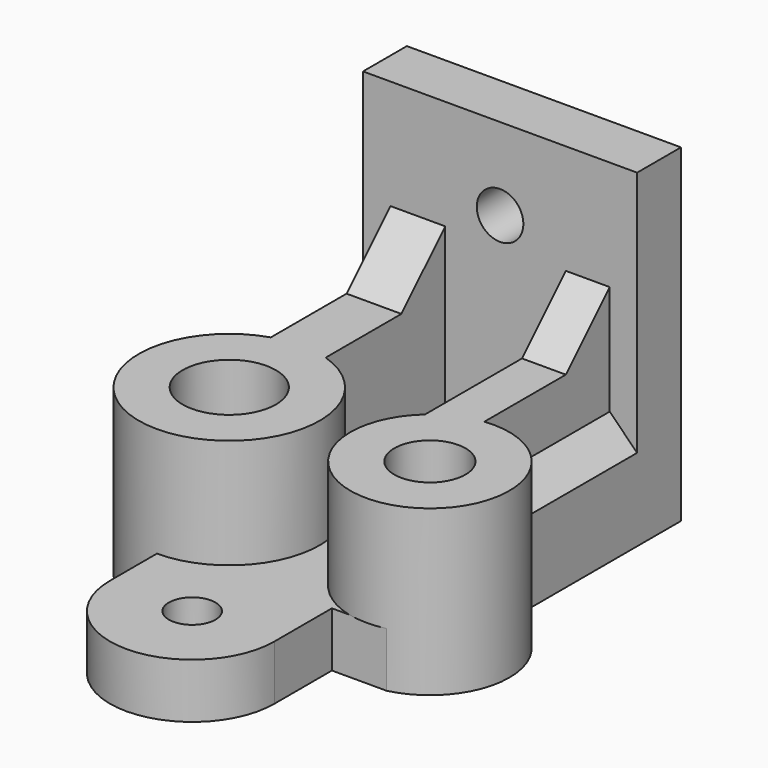
from build123d import *

# Parameters (mm, degrees)
F0_R          = 2.125
F0_R_2        = 4.25
F0_R_3        = 3.25
F1_DEPTH      = 5
F2_W          = 25
F2_H          = 5
F3_DEPTH      = 25
F4_R          = 8.25
F4_R_2        = 4.25
F4_R_3        = 7.25
F4_R_4        = 3.25
F5_DEPTH      = 10
F6_R          = 2.125
F7_DEPTH      = 5.001
F8_W          = 5
F8_H          = 13.6379074032
F8_W_2        = 4
F8_H_2        = 16.0665388563
F9_DEPTH      = 10
F10_T1_DEPTH  = 5
F10_T3_DEPTH  = 4
F10_T8_DEPTH  = 17.8584149398
F10_T13_DEPTH = 16.8584149398
F10_T18_DEPTH = 26.4963223431
F10_S19_R     = 8.25
F10_T20_DEPTH = 15
F10_T25_DEPTH = 26.4963223431
F10_S26_R     = 8.25
F10_T27_DEPTH = 15
F10_T32_DEPTH = 27.1526880508
F10_S34_R     = 7.25
F10_T35_DEPTH = 16


# Not quite as in the source:
# - a fillet or chamfer that OpenCascade refuses, or shapes differently, is made with other operations: its cross-section is extruded or revolved along the edge and cut away or added


with BuildPart() as f1:
    # F0 (on Top) → F1 (new body)
    with BuildSketch(Plane.XY):
        with BuildLine():
            Line((12.5, 26.5), (0, 26.5))
            Line((0, 26.5), (-12.5, 26.5))
            Line((-12.5, 26.5), (-12.5, 6.5622023742))
            ThreePointArc((-12.5, 6.5622023742), (-15.3166703137, -2.6385915194), (-7.5, -8.25))
            Line((-7.5, -8.25), (-7.5, -13.6))
            ThreePointArc((-7.5, -13.6), (-5.3033008589, -18.9033008589), (0, -21.1))
            ThreePointArc((0, -21.1), (5.3033008589, -18.9033008589), (7.5, -13.6))
            Line((7.5, -13.6), (7.5, -7.0478720193))
            Line((7.5, -7.0478720193), (12.5, -7.0478720193))
            ThreePointArc((12.5, -7.0478720193), (18.05, 0), (12.5, 7.0478720193))
            Line((12.5, 7.0478720193), (12.5, 26.5))
        make_face()
        with Locations((0, -13.6)):
            Circle(F0_R, mode=Mode.SUBTRACT)
        with Locations((-7.5, 0)):
            Circle(F0_R_2, mode=Mode.SUBTRACT)
        with Locations((10.8, 0)):
            Circle(F0_R_3, mode=Mode.SUBTRACT)
        with Locations((0, 16.5)):
            Circle(F0_R, mode=Mode.SUBTRACT)
    extrude(amount=F1_DEPTH)

    # F2 (on face) → F3 (join)
    with BuildSketch(Plane.XY.offset(5)):
        with Locations((0, 24)):
            Rectangle(F2_W, F2_H)
    extrude(amount=F3_DEPTH)

    # F4 (on face) → F5 (join)
    with BuildSketch(Plane.XY.offset(5)):
        with Locations((-7.5, 0)):
            Circle(F4_R)
        with Locations((-7.5, 0)):
            Circle(F4_R_2, mode=Mode.SUBTRACT)
        with Locations((10.8, 0)):
            Circle(F4_R_3)
        with Locations((10.8, 0)):
            Circle(F4_R_4, mode=Mode.SUBTRACT)
    extrude(amount=F5_DEPTH)

    # F6 (on face) → F7 (cut, through all)
    with BuildSketch(Plane.XZ.offset(-21.5)):
        with Locations((0, 22.5)):
            Circle(F6_R)
    extrude(amount=-F7_DEPTH, mode=Mode.SUBTRACT)

    # F8 (on face) → F9 (join)
    with BuildSketch(Plane.XY.offset(5)):
        with Locations((-7.5, 14.6810462984)):
            Rectangle(F8_W, F8_H)
        with Locations((8, 13.4667305718)):
            Rectangle(F8_W_2, F8_H_2)
    extrude(amount=F9_DEPTH)

    # F10: chamfer of 5 on 4 edges, made by hand

    # F10_s2 → F10_t1 (join)
    with BuildSketch(Plane.YZ.offset(-10)):
        Polygon((16.5, 15), (21.5, 20), (21.5, 15), align=None)
    extrude(amount=F10_T1_DEPTH)

    # F10_s4 → F10_t3 (join)
    with BuildSketch(Plane.YZ.offset(6)):
        Polygon((16.5, 15), (21.5, 20), (21.5, 15), align=None)
    extrude(amount=F10_T3_DEPTH)


with BuildPart() as f10_tool6:
    # F10_s7 → F10_t8 (new body)
    with BuildSketch(Plane.YZ.offset(7.8584149398)):
        Polygon((16.5, 15), (21.5, 20), (21.5, 15), align=None)
    extrude(amount=-F10_T8_DEPTH)

    split(bisect_by=Plane.YZ.offset(6), keep=Keep.TOP)


with BuildPart() as f1_1:
    add(f1.part)

    # F10_t5: union F10_tool6
    add(f10_tool6.part)


with BuildPart() as f10_tool11:
    # F10_s12 → F10_t13 (new body)
    with BuildSketch(Plane.YZ.offset(10)):
        Polygon((16.5, 15), (21.5, 20), (21.5, 15), align=None)
    extrude(amount=-F10_T13_DEPTH)

    split(bisect_by=Plane.YZ.offset(-5), keep=Keep.BOTTOM)


with BuildPart() as f1_2:
    add(f1_1.part)

    # F10_t10: union F10_tool11
    add(f10_tool11.part)


with BuildPart() as f10_tool16:
    # F10_s17 → F10_t18 (new body)
    with BuildSketch(Plane.XZ.offset(-21.5)):
        Polygon((-10, 10), (-15, 5), (-10, 5), align=None)
    extrude(amount=F10_T18_DEPTH)

    # F10_s19 → F10_t20 (cut, symmetric)
    with BuildSketch(Plane.XY.offset(7.5)):
        with Locations((-7.5, 0)):
            Circle(F10_S19_R)
    extrude(amount=F10_T20_DEPTH, both=True, mode=Mode.SUBTRACT)

    split(bisect_by=Plane.YZ.offset(-12.5), keep=Keep.TOP)


with BuildPart() as f1_3:
    add(f1_2.part)

    # F10_t15: union F10_tool16
    add(f10_tool16.part)


with BuildPart() as f10_tool23:
    # F10_s24 → F10_t25 (new body)
    with BuildSketch(Plane.XZ.offset(-21.5)):
        Polygon((-10, 10), (-15, 5), (-10, 5), align=None)
    extrude(amount=F10_T25_DEPTH)

    # F10_s26 → F10_t27 (intersect, symmetric)
    with BuildSketch(Plane.XY.offset(7.5)):
        with Locations((-7.5, 0)):
            Circle(F10_S26_R)
    extrude(amount=F10_T27_DEPTH, both=True, mode=Mode.INTERSECT)

    split(bisect_by=Plane.YZ.offset(-12.5), keep=Keep.BOTTOM)


with BuildPart() as f1_4:
    add(f1_3.part)

    # F10_t22: union F10_tool23
    add(f10_tool23.part)


with BuildPart() as f10_tool30:
    # F10_s31 → F10_t32 (new body)
    with BuildSketch(Plane.XZ.offset(5.6526880508)):
        Polygon((10, 10), (15, 5), (10, 5), align=None)
    extrude(amount=-F10_T32_DEPTH)

    split(bisect_by=Plane.YZ.offset(12.5), keep=Keep.BOTTOM)

    # F10_s34 → F10_t35 (cut, symmetric)
    with BuildSketch(Plane.XY.offset(7.5)):
        with Locations((10.8, 0)):
            Circle(F10_S34_R)
    extrude(amount=F10_T35_DEPTH, both=True, mode=Mode.SUBTRACT)


with BuildPart() as f1_5:
    add(f1_4.part)

    # F10_t29: union F10_tool30
    add(f10_tool30.part)


solid = f1_5.part
